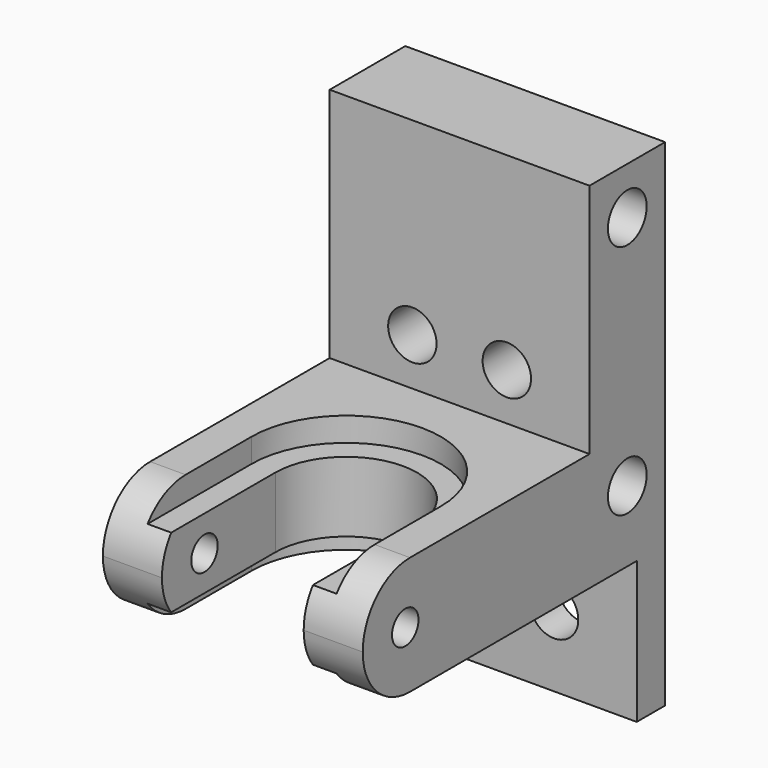
from build123d import *

# Parameters (mm, degrees)
F0_W     = 22
F0_H     = 42
F1_DEPTH = 3
F2_W     = 3
F2_H     = 30
F2_W_2   = 5
F3_DEPTH = 22
F4_D     = 4.1
F7_DEPTH = 5
F8_DEPTH = 2.97
F9_R     = 4.99999
F11_D    = 4.1
F12_D    = 2.8


# Not quite as in the source:
# - a fillet or chamfer is up to 0.001 mm smaller than in the source, because OpenCascade refuses the exact size


with BuildPart() as f1:
    # F0 (on Front) → F1 (new body)
    with BuildSketch(Plane.XZ):
        with Locations((-28.9233987555, 27.9422005266)):
            Rectangle(F0_W, F0_H)
    extrude(amount=F1_DEPTH)

    # F2 (on face) → F3 (join)
    with BuildSketch(Plane(origin=(-39.9233987555, 0, 0), x_dir=(0, -1, 0), z_dir=(-1, 0, 0))):
        with Locations((1.5, 33.9422005266)):
            Rectangle(F2_W, F2_H)
        with Locations((5.5, 33.9422005266)):
            Rectangle(F2_W_2, F2_H)
    extrude(amount=-F3_DEPTH)

    # F4 (through all)
    with Locations(Plane(origin=(0, 0, 0), x_dir=(1, 0, 0), z_dir=(0, 1, 0))):
        with Locations((-24.9233987555, -12.9422005266), (-32.9233987555, -12.9422005266), (-32.9233987555, -32.9422005266), (-24.9233987555, -32.9422005266)):
            Hole(F4_D / 2)

    # F6 (on line) → F7 (join, symmetric)
    with BuildSketch(Plane.XY.offset(23.9422005266)):
        with BuildLine():
            ThreePointArc((-36.9233987555, -20), (-28.9233987555, -12), (-20.9233987555, -20))
            Line((-20.9233987555, -20), (-20.9233987555, -32))
            Line((-20.9233987555, -32), (-17.9233987555, -32))
            Line((-17.9233987555, -32), (-17.9233987555, 0))
            Line((-17.9233987555, 0), (-39.9233987555, 0))
            Line((-39.9233987555, 0), (-39.9233987555, -32))
            Line((-39.9233987555, -32), (-36.9233987555, -32))
            Line((-36.9233987555, -32), (-36.9233987555, -20))
        make_face()
    extrude(amount=F7_DEPTH, both=True)

    # F6 (on line) → F8 (join, symmetric)
    with BuildSketch(Plane.XY.offset(23.9422005266)):
        with BuildLine():
            ThreePointArc((-34.9233987555, -20), (-28.9233987555, -14), (-22.9233987555, -20))
            Line((-22.9233987555, -20), (-22.9233987555, -25.2915026221))
            ThreePointArc((-22.9233987555, -25.2915026221), (-21.4400839819, -22.8284271247), (-20.9233987555, -20))
            ThreePointArc((-20.9233987555, -20), (-28.9233987555, -12), (-36.9233987555, -20))
            ThreePointArc((-36.9233987555, -20), (-36.406713529, -22.8284271247), (-34.9233987555, -25.2915026221))
            Line((-34.9233987555, -25.2915026221), (-34.9233987555, -20))
        make_face()
        with BuildLine():
            Line((-34.9233987555, -32), (-34.9233987555, -25.2915026221))
            ThreePointArc((-34.9233987555, -25.2915026221), (-36.406713529, -22.8284271247), (-36.9233987555, -20))
            Line((-36.9233987555, -20), (-36.9233987555, -32))
            Line((-36.9233987555, -32), (-34.9233987555, -32))
        make_face()
        with BuildLine():
            ThreePointArc((-20.9233987555, -20), (-21.4400839819, -22.8284271247), (-22.9233987555, -25.2915026221))
            Line((-22.9233987555, -25.2915026221), (-22.9233987555, -32))
            Line((-22.9233987555, -32), (-20.9233987555, -32))
            Line((-20.9233987555, -32), (-20.9233987555, -20))
        make_face()
    extrude(amount=F8_DEPTH, both=True)

    # F9 (radius 5 in the source; OpenCascade refuses exactly that, so slightly less here)
    f9_edges = [f1.edges().sort_by_distance(p)[0] for p in [
        (-38.423399, -32, 28.942201),
        (-38.423399, -32, 18.942201),
        (-19.423399, -32, 18.942201),
        (-19.423399, -32, 28.942201),
    ]]
    fillet(f9_edges, radius=F9_R)

    # F11 (through all)
    with Locations(Plane(origin=(-39.9233987555, 0, 0), x_dir=(0, -1, 0), z_dir=(-1, 0, 0))):
        with Locations((4, 44.9422005266), (4, 24.9422005266)):
            Hole(F11_D / 2)

    # F12 (through all)
    with Locations(Plane(origin=(-39.9233987555, 0, 0), x_dir=(0, -1, 0), z_dir=(-1, 0, 0))):
        with Locations((27.5, 23.9422005266)):
            Hole(F12_D / 2)


solid = f1.part
